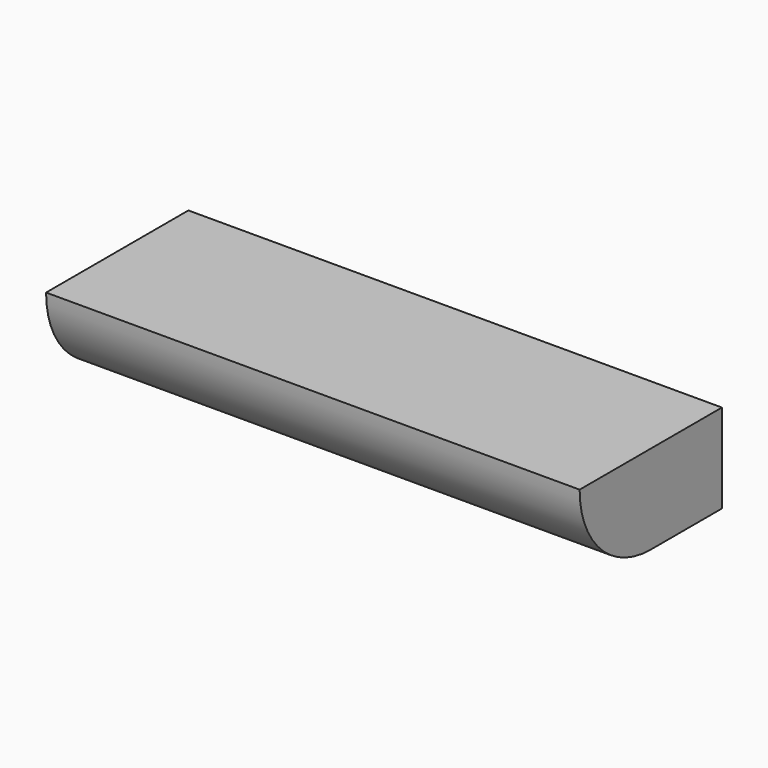
from build123d import *

# Parameters (mm, degrees)
F0_W     = 457.2
F0_H     = 76.2
F1_DEPTH = 152.4
F2_R     = 76.19999


# Not quite as in the source:
# - a fillet or chamfer is up to 0.001 mm smaller than in the source, because OpenCascade refuses the exact size


with BuildPart() as f1:
    # F0 (on Front) → F1 (new body)
    with BuildSketch(Plane.XZ):
        with Locations((20.4558894038, 8.9659971736)):
            Rectangle(F0_W, F0_H)
    extrude(amount=F1_DEPTH)

    # F2 (radius 76.2 in the source; OpenCascade refuses exactly that, so slightly less here)
    f2_edges = [f1.edges().sort_by_distance(p)[0] for p in [
        (20.455889, -152.4, -29.134003),
    ]]
    fillet(f2_edges, radius=F2_R)


solid = f1.part
